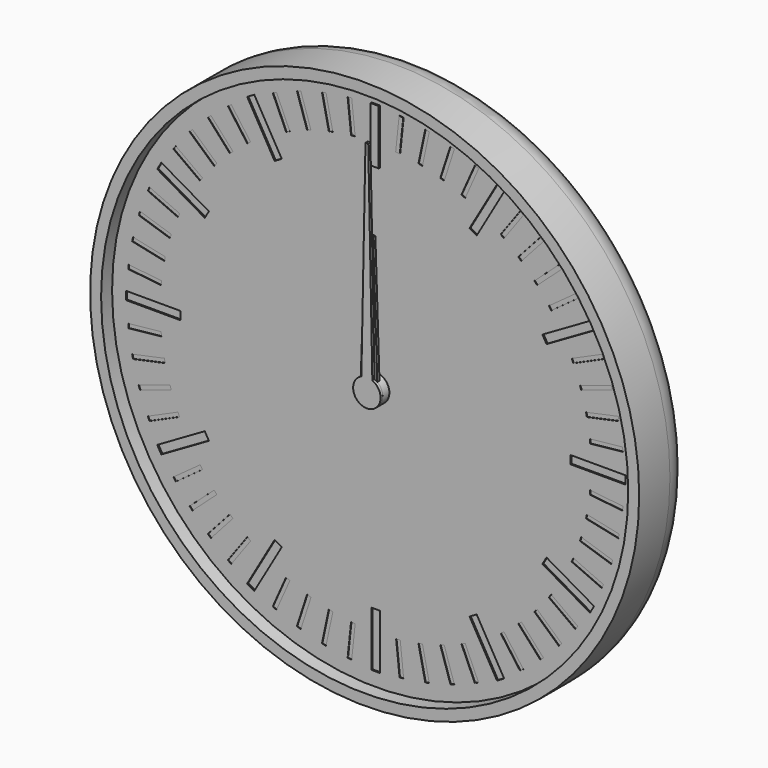
from build123d import *

# Parameters (mm, degrees)
F0_R      = 100
F1_DEPTH  = 24
F2_R      = 10
F3_T      = -4
F4_R      = 5
F4_R_2    = 3
F5_DEPTH  = 2
F6_DEPTH  = 19
F7_DEPTH  = 8
F9_DEPTH  = 4
F11_DEPTH = 4
F12_R     = 5
F12_R_2   = 3
F13_DEPTH = 2
F14_R     = 3
F15_DEPTH = 4
F17_DEPTH = 4
F18_R     = 3
F19_DEPTH = 2
F20_R     = 98
F20_R_2   = 5
F21_DEPTH = 1
F23_R     = 5
F23_R_2   = 3
F24_DEPTH = 2
F25_W     = 3
F25_H     = 20
F25_W_2   = 20
F25_H_2   = 3
F26_DEPTH = 0.5
F27_W     = 1.5
F27_H     = 12
F27_W_2   = 12
F27_H_2   = 1.5
F28_DEPTH = 0.2
F29_DEPTH = 1
F30_DEPTH = 0.4
F31_R     = 5
F31_R_2   = 3
F32_DEPTH = 5
F33_R     = 3
F34_DEPTH = 1
F36_DEPTH = 1


with BuildPart() as f1:
    # F0 (on Front) → F1 (new body)
    with BuildSketch(Plane.XZ):
        Circle(F0_R)
    extrude(amount=F1_DEPTH)

    # F2
    f2_edges = [f1.edges().sort_by_distance(p)[0] for p in [
        (-100, 0, 0),
    ]]
    fillet(f2_edges, radius=F2_R)

    # F3
    f3_openings = [f1.faces().sort_by_distance(p)[0] for p in [
        (0, -24, 0),
    ]]
    offset(amount=F3_T, openings=f3_openings)

    # F4 (on face) → F5 (join)
    with BuildSketch(Plane.XZ.offset(4)):
        Circle(F4_R)
        Circle(F4_R_2, mode=Mode.SUBTRACT)
        with Locations((40, 0)):
            Circle(F4_R)
        with Locations((40, 0)):
            Circle(F4_R_2, mode=Mode.SUBTRACT)
    extrude(amount=F5_DEPTH)


with BuildPart() as f6:
    # F6 (new): a face of the model
    f6_faces = [f1.part.faces().sort_by_distance(p)[0] for p in [
        (0, -4, 0),
    ]]
    extrude(f6_faces, amount=F6_DEPTH)

    # F8 (on face) → F9 (join)
    with BuildSketch(Plane.XZ.offset(6)):
        with BuildLine():
            ThreePointArc((9.2729637667, -1.3794085621), (9.3494561423, -0.6915886375), (9.375, 0))
            ThreePointArc((9.375, 0), (9.3494561423, 0.6915886375), (9.2729637667, 1.3794085621))
            ThreePointArc((9.2729637667, 1.3794085621), (8.9161548403, 2.8970343223), (8.3127812852, 4.3345463782))
            ThreePointArc((8.3127812852, 4.3345463782), (7.5845343223, 5.5104867402), (6.6911892658, 6.566476316))
            ThreePointArc((6.6911892658, 6.566476316), (5.5104867402, 7.5845343223), (4.1773988938, 8.3928519278))
            ThreePointArc((4.1773988938, 8.3928519278), (2.8970343223, 8.9161548403), (1.5536078905, 9.2453733036))
            ThreePointArc((1.5536078905, 9.2453733036), (0, 9.375), (-1.5536078905, 9.2453733036))
            ThreePointArc((-1.5536078905, 9.2453733036), (-2.8970343223, 8.9161548403), (-4.1773988938, 8.3928519278))
            ThreePointArc((-4.1773988938, 8.3928519278), (-5.5104867402, 7.5845343223), (-6.6911892658, 6.566476316))
            ThreePointArc((-6.6911892658, 6.566476316), (-7.5845343223, 5.5104867402), (-8.3127812852, 4.3345463782))
            ThreePointArc((-8.3127812852, 4.3345463782), (-8.9161548403, 2.8970343223), (-9.2729637667, 1.3794085621))
            ThreePointArc((-9.2729637667, 1.3794085621), (-9.375, 0), (-9.2729637667, -1.3794085621))
            ThreePointArc((-9.2729637667, -1.3794085621), (-8.9161548403, -2.8970343223), (-8.3127812852, -4.3345463782))
            ThreePointArc((-8.3127812852, -4.3345463782), (-7.5845343223, -5.5104867402), (-6.6911892658, -6.566476316))
            ThreePointArc((-6.6911892658, -6.566476316), (-5.5104867402, -7.5845343223), (-4.1773988938, -8.3928519278))
            ThreePointArc((-4.1773988938, -8.3928519278), (-2.8970343223, -8.9161548403), (-1.5536078905, -9.2453733036))
            ThreePointArc((-1.5536078905, -9.2453733036), (0, -9.375), (1.5536078905, -9.2453733036))
            ThreePointArc((1.5536078905, -9.2453733036), (2.8970343223, -8.9161548403), (4.1773988938, -8.3928519278))
            ThreePointArc((4.1773988938, -8.3928519278), (5.5104867402, -7.5845343223), (6.6911892658, -6.566476316))
            ThreePointArc((6.6911892658, -6.566476316), (7.5845343223, -5.5104867402), (8.3127812852, -4.3345463782))
            ThreePointArc((8.3127812852, -4.3345463782), (8.9161548403, -2.8970343223), (9.2729637667, -1.3794085621))
        make_face()
        with BuildLine():
            ThreePointArc((8.3127812852, 4.3345463782), (8.9161548403, 2.8970343223), (9.2729637667, 1.3794085621))
            Line((9.2729637667, 1.3794085621), (11.1823199426, 2.3946312492))
            Line((11.1823199426, 2.3946312492), (10.8182678729, 3.515068311))
            Line((10.8182678729, 3.515068311), (10.4542158031, 4.6355053728))
            Line((10.4542158031, 4.6355053728), (8.3127812852, 4.3345463782))
        make_face()
        with BuildLine():
            Line((11.1823199426, -2.3946312492), (9.2729637667, -1.3794085621))
            ThreePointArc((9.2729637667, -1.3794085621), (8.9161548403, -2.8970343223), (8.3127812852, -4.3345463782))
            Line((8.3127812852, -4.3345463782), (10.4542158031, -4.6355053728))
            Line((10.4542158031, -4.6355053728), (10.8182678729, -3.515068311))
            Line((10.8182678729, -3.515068311), (11.1823199426, -2.3946312492))
        make_face()
        with BuildLine():
            ThreePointArc((4.1773988938, 8.3928519278), (5.5104867402, 7.5845343223), (6.6911892658, 6.566476316))
            Line((6.6911892658, 6.566476316), (7.6391579371, 8.5101001246))
            Line((7.6391579371, 8.5101001246), (6.6860572448, 9.202568311))
            Line((6.6860572448, 9.202568311), (5.7329565525, 9.8950364974))
            Line((5.7329565525, 9.8950364974), (4.1773988938, 8.3928519278))
        make_face()
        with BuildLine():
            Line((7.6391579371, -8.5101001246), (6.6911892658, -6.566476316))
            ThreePointArc((6.6911892658, -6.566476316), (5.5104867402, -7.5845343223), (4.1773988938, -8.3928519278))
            Line((4.1773988938, -8.3928519278), (5.7329565525, -9.8950364974))
            Line((5.7329565525, -9.8950364974), (6.6860572448, -9.202568311))
            Line((6.6860572448, -9.202568311), (7.6391579371, -8.5101001246))
        make_face()
        with BuildLine():
            ThreePointArc((-1.5536078905, 9.2453733036), (0, 9.375), (1.5536078905, 9.2453733036))
            Line((1.5536078905, 9.2453733036), (1.1780972451, 11.375))
            Line((1.1780972451, 11.375), (0, 11.375))
            Line((0, 11.375), (-1.1780972451, 11.375))
            Line((-1.1780972451, 11.375), (-1.5536078905, 9.2453733036))
        make_face()
        with BuildLine():
            Line((1.1780972451, -11.375), (1.5536078905, -9.2453733036))
            ThreePointArc((1.5536078905, -9.2453733036), (0, -9.375), (-1.5536078905, -9.2453733036))
            Line((-1.5536078905, -9.2453733036), (-1.1780972451, -11.375))
            Line((-1.1780972451, -11.375), (0, -11.375))
            Line((0, -11.375), (1.1780972451, -11.375))
        make_face()
        with BuildLine():
            ThreePointArc((-6.6911892658, 6.566476316), (-5.5104867402, 7.5845343223), (-4.1773988938, 8.3928519278))
            Line((-4.1773988938, 8.3928519278), (-5.7329565525, 9.8950364974))
            Line((-5.7329565525, 9.8950364974), (-6.6860572448, 9.202568311))
            Line((-6.6860572448, 9.202568311), (-7.6391579371, 8.5101001246))
            Line((-7.6391579371, 8.5101001246), (-6.6911892658, 6.566476316))
        make_face()
        with BuildLine():
            Line((-5.7329565525, -9.8950364974), (-4.1773988938, -8.3928519278))
            ThreePointArc((-4.1773988938, -8.3928519278), (-5.5104867402, -7.5845343223), (-6.6911892658, -6.566476316))
            Line((-6.6911892658, -6.566476316), (-7.6391579371, -8.5101001246))
            Line((-7.6391579371, -8.5101001246), (-6.6860572448, -9.202568311))
            Line((-6.6860572448, -9.202568311), (-5.7329565525, -9.8950364974))
        make_face()
        with BuildLine():
            ThreePointArc((-9.2729637667, 1.3794085621), (-8.9161548403, 2.8970343223), (-8.3127812852, 4.3345463782))
            Line((-8.3127812852, 4.3345463782), (-10.4542158031, 4.6355053728))
            Line((-10.4542158031, 4.6355053728), (-10.8182678729, 3.515068311))
            Line((-10.8182678729, 3.515068311), (-11.1823199426, 2.3946312492))
            Line((-11.1823199426, 2.3946312492), (-9.2729637667, 1.3794085621))
        make_face()
        with BuildLine():
            Line((-10.4542158031, -4.6355053728), (-8.3127812852, -4.3345463782))
            ThreePointArc((-8.3127812852, -4.3345463782), (-8.9161548403, -2.8970343223), (-9.2729637667, -1.3794085621))
            Line((-9.2729637667, -1.3794085621), (-11.1823199426, -2.3946312492))
            Line((-11.1823199426, -2.3946312492), (-10.8182678729, -3.515068311))
            Line((-10.8182678729, -3.515068311), (-10.4542158031, -4.6355053728))
        make_face()
    extrude(amount=F9_DEPTH)

    # F35 (on face) → F36 (join)
    with BuildSketch(Plane.XZ.offset(23)):
        with BuildLine():
            ThreePointArc((-2, 4.582575695), (-2.7386127875, -4.1833001327), (5, 0))
            ThreePointArc((5, 0), (4.1833001327, 2.7386127875), (2, 4.582575695))
            ThreePointArc((2, 4.582575695), (0, 5), (-2, 4.582575695))
        make_face()
        with BuildLine():
            ThreePointArc((-2, 4.582575695), (0, 5), (2, 4.582575695))
            Line((2, 4.582575695), (0.5, 80))
            Line((0.5, 80), (0, 80))
            Line((0, 80), (-0.5, 80))
            Line((-0.5, 80), (-2, 4.582575695))
        make_face()
    extrude(amount=-F36_DEPTH)


with BuildPart() as f7:
    # F7 (new): a face of the model
    f7_faces = [f1.part.faces().sort_by_distance(p)[0] for p in [
        (40, -4, 0),
    ]]
    extrude(f7_faces, amount=F7_DEPTH)

    # F10 (on face) → F11 (join)
    with BuildSketch(Plane.XZ.offset(6)):
        with BuildLine():
            ThreePointArc((68.0829066802, -1.5381733945), (68.1144747006, -0.7693746225), (68.125, 0))
            ThreePointArc((68.125, 0), (68.1144747006, 0.7693746225), (68.0829066802, 1.5381733945))
            ThreePointArc((68.0829066802, 1.5381733945), (67.9709283072, 2.9398630294), (67.7890320221, 4.3342039956))
            ThreePointArc((67.7890320221, 4.3342039956), (67.5104012706, 5.8475163042), (67.1494235596, 7.3433252263))
            ThreePointArc((67.1494235596, 7.3433252263), (66.7484645208, 8.6911029668), (66.280643318, 10.0171558733))
            ThreePointArc((66.280643318, 10.0171558733), (65.6934659962, 11.4394680865), (65.0293803521, 12.8275385085))
            ThreePointArc((65.0293803521, 12.8275385085), (64.3569644814, 14.0625), (63.6236643925, 15.2623099717))
            ThreePointArc((63.6236643925, 15.2623099717), (62.7536029668, 16.5314602207), (61.815433119, 17.7511268046))
            ThreePointArc((61.815433119, 17.7511268046), (60.9009482166, 18.8192983038), (59.934217974, 19.8404278876))
            ThreePointArc((59.934217974, 19.8404278876), (58.8192983038, 20.9009482166), (57.6480467764, 21.8989056799))
            ThreePointArc((57.6480467764, 21.8989056799), (56.5314602207, 22.7536029668), (55.3735505752, 23.5514238999))
            ThreePointArc((55.3735505752, 23.5514238999), (54.0625, 24.3569644814), (52.709356105, 25.0895972944))
            ThreePointArc((52.709356105, 25.0895972944), (51.4394680865, 25.6934659962), (50.1409852457, 26.2331096755))
            ThreePointArc((50.1409852457, 26.2331096755), (48.6911029668, 26.7484645208), (47.2152055856, 27.1837531139))
            ThreePointArc((47.2152055856, 27.1837531139), (45.8475163042, 27.5104012706), (44.4652101991, 27.7682826779))
            ThreePointArc((44.4652101991, 27.7682826779), (42.9398630294, 27.9709283072), (41.4057159597, 28.0898484802))
            ThreePointArc((41.4057159597, 28.0898484802), (40, 28.125), (38.5942840403, 28.0898484802))
            ThreePointArc((38.5942840403, 28.0898484802), (37.0601369706, 27.9709283072), (35.5347898009, 27.7682826779))
            ThreePointArc((35.5347898009, 27.7682826779), (34.1524836958, 27.5104012706), (32.7847944144, 27.1837531139))
            ThreePointArc((32.7847944144, 27.1837531139), (31.3088970332, 26.7484645208), (29.8590147543, 26.2331096755))
            ThreePointArc((29.8590147543, 26.2331096755), (28.5605319135, 25.6934659962), (27.290643895, 25.0895972944))
            ThreePointArc((27.290643895, 25.0895972944), (25.9375, 24.3569644814), (24.6264494248, 23.5514238999))
            ThreePointArc((24.6264494248, 23.5514238999), (23.4685397793, 22.7536029668), (22.3519532236, 21.8989056799))
            ThreePointArc((22.3519532236, 21.8989056799), (21.1807016962, 20.9009482166), (20.065782026, 19.8404278876))
            ThreePointArc((20.065782026, 19.8404278876), (19.0990517834, 18.8192983038), (18.184566881, 17.7511268046))
            ThreePointArc((18.184566881, 17.7511268046), (17.2463970332, 16.5314602207), (16.3763356075, 15.2623099717))
            ThreePointArc((16.3763356075, 15.2623099717), (15.6430355186, 14.0625), (14.9706196479, 12.8275385085))
            ThreePointArc((14.9706196479, 12.8275385085), (14.3065340038, 11.4394680865), (13.719356682, 10.0171558733))
            ThreePointArc((13.719356682, 10.0171558733), (13.2515354792, 8.6911029668), (12.8505764404, 7.3433252263))
            ThreePointArc((12.8505764404, 7.3433252263), (12.4895987294, 5.8475163042), (12.2109679779, 4.3342039956))
            ThreePointArc((12.2109679779, 4.3342039956), (12.0290716928, 2.9398630294), (11.9170933198, 1.5381733945))
            ThreePointArc((11.9170933198, 1.5381733945), (11.875, 0), (11.9170933198, -1.5381733945))
            ThreePointArc((11.9170933198, -1.5381733945), (12.0290716928, -2.9398630294), (12.2109679779, -4.3342039956))
            ThreePointArc((12.2109679779, -4.3342039956), (12.4895987294, -5.8475163042), (12.8505764404, -7.3433252263))
            ThreePointArc((12.8505764404, -7.3433252263), (13.2515354792, -8.6911029668), (13.719356682, -10.0171558733))
            ThreePointArc((13.719356682, -10.0171558733), (14.3065340038, -11.4394680865), (14.9706196479, -12.8275385085))
            ThreePointArc((14.9706196479, -12.8275385085), (15.6430355186, -14.0625), (16.3763356075, -15.2623099717))
            ThreePointArc((16.3763356075, -15.2623099717), (17.2463970332, -16.5314602207), (18.184566881, -17.7511268046))
            ThreePointArc((18.184566881, -17.7511268046), (19.0990517834, -18.8192983038), (20.065782026, -19.8404278876))
            ThreePointArc((20.065782026, -19.8404278876), (21.1807016962, -20.9009482166), (22.3519532236, -21.8989056799))
            ThreePointArc((22.3519532236, -21.8989056799), (23.4685397793, -22.7536029668), (24.6264494248, -23.5514238999))
            ThreePointArc((24.6264494248, -23.5514238999), (25.9375, -24.3569644814), (27.290643895, -25.0895972944))
            ThreePointArc((27.290643895, -25.0895972944), (28.5605319135, -25.6934659962), (29.8590147543, -26.2331096755))
            ThreePointArc((29.8590147543, -26.2331096755), (31.3088970332, -26.7484645208), (32.7847944144, -27.1837531139))
            ThreePointArc((32.7847944144, -27.1837531139), (34.1524836958, -27.5104012706), (35.5347898009, -27.7682826779))
            ThreePointArc((35.5347898009, -27.7682826779), (37.0601369706, -27.9709283072), (38.5942840403, -28.0898484802))
            ThreePointArc((38.5942840403, -28.0898484802), (40, -28.125), (41.4057159597, -28.0898484802))
            ThreePointArc((41.4057159597, -28.0898484802), (42.9398630294, -27.9709283072), (44.4652101991, -27.7682826779))
            ThreePointArc((44.4652101991, -27.7682826779), (45.8475163042, -27.5104012706), (47.2152055856, -27.1837531139))
            ThreePointArc((47.2152055856, -27.1837531139), (48.6911029668, -26.7484645208), (50.1409852457, -26.2331096755))
            ThreePointArc((50.1409852457, -26.2331096755), (51.4394680865, -25.6934659962), (52.709356105, -25.0895972944))
            ThreePointArc((52.709356105, -25.0895972944), (54.0625, -24.3569644814), (55.3735505752, -23.5514238999))
            ThreePointArc((55.3735505752, -23.5514238999), (56.5314602207, -22.7536029668), (57.6480467764, -21.8989056799))
            ThreePointArc((57.6480467764, -21.8989056799), (58.8192983038, -20.9009482166), (59.934217974, -19.8404278876))
            ThreePointArc((59.934217974, -19.8404278876), (60.9009482166, -18.8192983038), (61.815433119, -17.7511268046))
            ThreePointArc((61.815433119, -17.7511268046), (62.7536029668, -16.5314602207), (63.6236643925, -15.2623099717))
            ThreePointArc((63.6236643925, -15.2623099717), (64.3569644814, -14.0625), (65.0293803521, -12.8275385085))
            ThreePointArc((65.0293803521, -12.8275385085), (65.6934659962, -11.4394680865), (66.280643318, -10.0171558733))
            ThreePointArc((66.280643318, -10.0171558733), (66.7484645208, -8.6911029668), (67.1494235596, -7.3433252263))
            ThreePointArc((67.1494235596, -7.3433252263), (67.5104012706, -5.8475163042), (67.7890320221, -4.3342039956))
            ThreePointArc((67.7890320221, -4.3342039956), (67.9709283072, -2.9398630294), (68.0829066802, -1.5381733945))
        make_face()
        with BuildLine():
            ThreePointArc((68.0829066802, 1.5381733945), (68.1144747006, 0.7693746225), (68.125, 0))
            ThreePointArc((68.125, 0), (68.1144747006, -0.7693746225), (68.0829066802, -1.5381733945))
            Line((68.0829066802, -1.5381733945), (70.125, -1.1780972451))
            Line((70.125, -1.1780972451), (70.125, 0))
            Line((70.125, 0), (70.125, 1.1780972451))
            Line((70.125, 1.1780972451), (68.0829066802, 1.5381733945))
        make_face()
        with BuildLine():
            ThreePointArc((67.1494235596, 7.3433252263), (67.5104012706, 5.8475163042), (67.7890320221, 4.3342039956))
            Line((67.7890320221, 4.3342039956), (69.7116366623, 5.1109866922))
            Line((69.7116366623, 5.1109866922), (69.4666964721, 6.2633396859))
            Line((69.4666964721, 6.2633396859), (69.2217562819, 7.4156926796))
            Line((69.2217562819, 7.4156926796), (67.1494235596, 7.3433252263))
        make_face()
        with BuildLine():
            Line((69.7116366623, -5.1109866922), (67.7890320221, -4.3342039956))
            ThreePointArc((67.7890320221, -4.3342039956), (67.5104012706, -5.8475163042), (67.1494235596, -7.3433252263))
            Line((67.1494235596, -7.3433252263), (69.2217562819, -7.4156926796))
            Line((69.2217562819, -7.4156926796), (69.4666964721, -6.2633396859))
            Line((69.4666964721, -6.2633396859), (69.7116366623, -5.1109866922))
        make_face()
        with BuildLine():
            ThreePointArc((65.0293803521, 12.8275385085), (65.6934659962, 11.4394680865), (66.280643318, 10.0171558733))
            Line((66.280643318, 10.0171558733), (67.9997322302, 11.1766959857))
            Line((67.9997322302, 11.1766959857), (67.5205569115, 12.2529413727))
            Line((67.5205569115, 12.2529413727), (67.0413815928, 13.3291867596))
            Line((67.0413815928, 13.3291867596), (65.0293803521, 12.8275385085))
        make_face()
        with BuildLine():
            Line((67.9997322302, -11.1766959857), (66.280643318, -10.0171558733))
            ThreePointArc((66.280643318, -10.0171558733), (65.6934659962, -11.4394680865), (65.0293803521, -12.8275385085))
            Line((65.0293803521, -12.8275385085), (67.0413815928, -13.3291867596))
            Line((67.0413815928, -13.3291867596), (67.5205569115, -12.2529413727))
            Line((67.5205569115, -12.2529413727), (67.9997322302, -11.1766959857))
        make_face()
        with BuildLine():
            ThreePointArc((61.815433119, 17.7511268046), (62.7536029668, 16.5314602207), (63.6236643925, 15.2623099717))
            Line((63.6236643925, 15.2623099717), (65.064105142, 16.753930033))
            Line((65.064105142, 16.753930033), (64.3716369555, 17.7070307253))
            Line((64.3716369555, 17.7070307253), (63.6791687691, 18.6601314176))
            Line((63.6791687691, 18.6601314176), (61.815433119, 17.7511268046))
        make_face()
        with BuildLine():
            Line((65.064105142, -16.753930033), (63.6236643925, -15.2623099717))
            ThreePointArc((63.6236643925, -15.2623099717), (62.7536029668, -16.5314602207), (61.815433119, -17.7511268046))
            Line((61.815433119, -17.7511268046), (63.6791687691, -18.6601314176))
            Line((63.6791687691, -18.6601314176), (64.3716369555, -17.7070307253))
            Line((64.3716369555, -17.7070307253), (65.064105142, -16.753930033))
        make_face()
        with BuildLine():
            ThreePointArc((57.6480467764, 21.8989056799), (58.8192983038, 20.9009482166), (59.934217974, 19.8404278876))
            Line((59.934217974, 19.8404278876), (61.0330563882, 21.5989369435))
            Line((61.0330563882, 21.5989369435), (60.1575595166, 22.3872378675))
            Line((60.1575595166, 22.3872378675), (59.282062645, 23.1755387915))
            Line((59.282062645, 23.1755387915), (57.6480467764, 21.8989056799))
        make_face()
        with BuildLine():
            Line((61.0330563882, -21.5989369435), (59.934217974, -19.8404278876))
            ThreePointArc((59.934217974, -19.8404278876), (58.8192983038, -20.9009482166), (57.6480467764, -21.8989056799))
            Line((57.6480467764, -21.8989056799), (59.282062645, -23.1755387915))
            Line((59.282062645, -23.1755387915), (60.1575595166, -22.3872378675))
            Line((60.1575595166, -22.3872378675), (61.0330563882, -21.5989369435))
        make_face()
        with BuildLine():
            ThreePointArc((52.709356105, 25.0895972944), (54.0625, 24.3569644814), (55.3735505752, 23.5514238999))
            Line((55.3735505752, 23.5514238999), (56.0827621424, 25.4999666665))
            Line((56.0827621424, 25.4999666665), (55.0625, 26.089015289))
            Line((55.0625, 26.089015289), (54.0422378576, 26.6780639116))
            Line((54.0422378576, 26.6780639116), (52.709356105, 25.0895972944))
        make_face()
        with BuildLine():
            Line((56.0827621424, -25.4999666665), (55.3735505752, -23.5514238999))
            ThreePointArc((55.3735505752, -23.5514238999), (54.0625, -24.3569644814), (52.709356105, -25.0895972944))
            Line((52.709356105, -25.0895972944), (54.0422378576, -26.6780639116))
            Line((54.0422378576, -26.6780639116), (55.0625, -26.089015289))
            Line((55.0625, -26.089015289), (56.0827621424, -25.4999666665))
        make_face()
        with BuildLine():
            ThreePointArc((47.2152055856, 27.1837531139), (48.6911029668, 26.7484645208), (50.1409852457, 26.2331096755))
            Line((50.1409852457, 26.2331096755), (50.4295740173, 28.2865254836))
            Line((50.4295740173, 28.2865254836), (49.3091369555, 28.6505775534))
            Line((49.3091369555, 28.6505775534), (48.1886998938, 29.0146296232))
            Line((48.1886998938, 29.0146296232), (47.2152055856, 27.1837531139))
        make_face()
        with BuildLine():
            Line((50.4295740173, -28.2865254836), (50.1409852457, -26.2331096755))
            ThreePointArc((50.1409852457, -26.2331096755), (48.6911029668, -26.7484645208), (47.2152055856, -27.1837531139))
            Line((47.2152055856, -27.1837531139), (48.1886998938, -29.0146296232))
            Line((48.1886998938, -29.0146296232), (49.3091369555, -28.6505775534))
            Line((49.3091369555, -28.6505775534), (50.4295740173, -28.2865254836))
        make_face()
        with BuildLine():
            ThreePointArc((41.4057159597, 28.0898484802), (42.9398630294, 27.9709283072), (44.4652101991, 27.7682826779))
            Line((44.4652101991, 27.7682826779), (44.3205634611, 29.8368274034))
            Line((44.3205634611, 29.8368274034), (43.1489199559, 29.959972098))
            Line((43.1489199559, 29.959972098), (41.9772764508, 30.0831167926))
            Line((41.9772764508, 30.0831167926), (41.4057159597, 28.0898484802))
        make_face()
        with BuildLine():
            Line((44.3205634611, -29.8368274034), (44.4652101991, -27.7682826779))
            ThreePointArc((44.4652101991, -27.7682826779), (42.9398630294, -27.9709283072), (41.4057159597, -28.0898484802))
            Line((41.4057159597, -28.0898484802), (41.9772764508, -30.0831167926))
            Line((41.9772764508, -30.0831167926), (43.1489199559, -29.959972098))
            Line((43.1489199559, -29.959972098), (44.3205634611, -29.8368274034))
        make_face()
        with BuildLine():
            ThreePointArc((35.5347898009, 27.7682826779), (37.0601369706, 27.9709283072), (38.5942840403, 28.0898484802))
            Line((38.5942840403, 28.0898484802), (38.0227235492, 30.0831167926))
            Line((38.0227235492, 30.0831167926), (36.8510800441, 29.959972098))
            Line((36.8510800441, 29.959972098), (35.6794365389, 29.8368274034))
            Line((35.6794365389, 29.8368274034), (35.5347898009, 27.7682826779))
        make_face()
        with BuildLine():
            Line((38.0227235492, -30.0831167926), (38.5942840403, -28.0898484802))
            ThreePointArc((38.5942840403, -28.0898484802), (37.0601369706, -27.9709283072), (35.5347898009, -27.7682826779))
            Line((35.5347898009, -27.7682826779), (35.6794365389, -29.8368274034))
            Line((35.6794365389, -29.8368274034), (36.8510800441, -29.959972098))
            Line((36.8510800441, -29.959972098), (38.0227235492, -30.0831167926))
        make_face()
        with BuildLine():
            ThreePointArc((29.8590147543, 26.2331096755), (31.3088970332, 26.7484645208), (32.7847944144, 27.1837531139))
            Line((32.7847944144, 27.1837531139), (31.8113001062, 29.0146296232))
            Line((31.8113001062, 29.0146296232), (30.6908630445, 28.6505775534))
            Line((30.6908630445, 28.6505775534), (29.5704259827, 28.2865254836))
            Line((29.5704259827, 28.2865254836), (29.8590147543, 26.2331096755))
        make_face()
        with BuildLine():
            Line((31.8113001062, -29.0146296232), (32.7847944144, -27.1837531139))
            ThreePointArc((32.7847944144, -27.1837531139), (31.3088970332, -26.7484645208), (29.8590147543, -26.2331096755))
            Line((29.8590147543, -26.2331096755), (29.5704259827, -28.2865254836))
            Line((29.5704259827, -28.2865254836), (30.6908630445, -28.6505775534))
            Line((30.6908630445, -28.6505775534), (31.8113001062, -29.0146296232))
        make_face()
        with BuildLine():
            ThreePointArc((24.6264494248, 23.5514238999), (25.9375, 24.3569644814), (27.290643895, 25.0895972944))
            Line((27.290643895, 25.0895972944), (25.9577621424, 26.6780639116))
            Line((25.9577621424, 26.6780639116), (24.9375, 26.089015289))
            Line((24.9375, 26.089015289), (23.9172378576, 25.4999666665))
            Line((23.9172378576, 25.4999666665), (24.6264494248, 23.5514238999))
        make_face()
        with BuildLine():
            Line((25.9577621424, -26.6780639116), (27.290643895, -25.0895972944))
            ThreePointArc((27.290643895, -25.0895972944), (25.9375, -24.3569644814), (24.6264494248, -23.5514238999))
            Line((24.6264494248, -23.5514238999), (23.9172378576, -25.4999666665))
            Line((23.9172378576, -25.4999666665), (24.9375, -26.089015289))
            Line((24.9375, -26.089015289), (25.9577621424, -26.6780639116))
        make_face()
        with BuildLine():
            ThreePointArc((20.065782026, 19.8404278876), (21.1807016962, 20.9009482166), (22.3519532236, 21.8989056799))
            Line((22.3519532236, 21.8989056799), (20.717937355, 23.1755387915))
            Line((20.717937355, 23.1755387915), (19.8424404834, 22.3872378675))
            Line((19.8424404834, 22.3872378675), (18.9669436118, 21.5989369435))
            Line((18.9669436118, 21.5989369435), (20.065782026, 19.8404278876))
        make_face()
        with BuildLine():
            Line((20.717937355, -23.1755387915), (22.3519532236, -21.8989056799))
            ThreePointArc((22.3519532236, -21.8989056799), (21.1807016962, -20.9009482166), (20.065782026, -19.8404278876))
            Line((20.065782026, -19.8404278876), (18.9669436118, -21.5989369435))
            Line((18.9669436118, -21.5989369435), (19.8424404834, -22.3872378675))
            Line((19.8424404834, -22.3872378675), (20.717937355, -23.1755387915))
        make_face()
        with BuildLine():
            ThreePointArc((16.3763356075, 15.2623099717), (17.2463970332, 16.5314602207), (18.184566881, 17.7511268046))
            Line((18.184566881, 17.7511268046), (16.3208312309, 18.6601314176))
            Line((16.3208312309, 18.6601314176), (15.6283630445, 17.7070307253))
            Line((15.6283630445, 17.7070307253), (14.935894858, 16.753930033))
            Line((14.935894858, 16.753930033), (16.3763356075, 15.2623099717))
        make_face()
        with BuildLine():
            Line((16.3208312309, -18.6601314176), (18.184566881, -17.7511268046))
            ThreePointArc((18.184566881, -17.7511268046), (17.2463970332, -16.5314602207), (16.3763356075, -15.2623099717))
            Line((16.3763356075, -15.2623099717), (14.935894858, -16.753930033))
            Line((14.935894858, -16.753930033), (15.6283630445, -17.7070307253))
            Line((15.6283630445, -17.7070307253), (16.3208312309, -18.6601314176))
        make_face()
        with BuildLine():
            ThreePointArc((13.719356682, 10.0171558733), (14.3065340038, 11.4394680865), (14.9706196479, 12.8275385085))
            Line((14.9706196479, 12.8275385085), (12.9586184072, 13.3291867596))
            Line((12.9586184072, 13.3291867596), (12.4794430885, 12.2529413727))
            Line((12.4794430885, 12.2529413727), (12.0002677698, 11.1766959857))
            Line((12.0002677698, 11.1766959857), (13.719356682, 10.0171558733))
        make_face()
        with BuildLine():
            Line((12.9586184072, -13.3291867596), (14.9706196479, -12.8275385085))
            ThreePointArc((14.9706196479, -12.8275385085), (14.3065340038, -11.4394680865), (13.719356682, -10.0171558733))
            Line((13.719356682, -10.0171558733), (12.0002677698, -11.1766959857))
            Line((12.0002677698, -11.1766959857), (12.4794430885, -12.2529413727))
            Line((12.4794430885, -12.2529413727), (12.9586184072, -13.3291867596))
        make_face()
        with BuildLine():
            ThreePointArc((12.2109679779, 4.3342039956), (12.4895987294, 5.8475163042), (12.8505764404, 7.3433252263))
            Line((12.8505764404, 7.3433252263), (10.7782437181, 7.4156926796))
            Line((10.7782437181, 7.4156926796), (10.5333035279, 6.2633396859))
            Line((10.5333035279, 6.2633396859), (10.2883633377, 5.1109866922))
            Line((10.2883633377, 5.1109866922), (12.2109679779, 4.3342039956))
        make_face()
        with BuildLine():
            Line((10.7782437181, -7.4156926796), (12.8505764404, -7.3433252263))
            ThreePointArc((12.8505764404, -7.3433252263), (12.4895987294, -5.8475163042), (12.2109679779, -4.3342039956))
            Line((12.2109679779, -4.3342039956), (10.2883633377, -5.1109866922))
            Line((10.2883633377, -5.1109866922), (10.5333035279, -6.2633396859))
            Line((10.5333035279, -6.2633396859), (10.7782437181, -7.4156926796))
        make_face()
        with BuildLine():
            ThreePointArc((11.9170933198, -1.5381733945), (11.875, 0), (11.9170933198, 1.5381733945))
            Line((11.9170933198, 1.5381733945), (9.875, 1.1780972451))
            Line((9.875, 1.1780972451), (9.875, 0))
            Line((9.875, 0), (9.875, -1.1780972451))
            Line((9.875, -1.1780972451), (11.9170933198, -1.5381733945))
        make_face()
    extrude(amount=F11_DEPTH)

    # F16 (on face) → F17 (join)
    with BuildSketch(Plane.XZ.offset(12)):
        with BuildLine():
            ThreePointArc((47.4288750323, -1.0304444454), (47.4821976298, -0.5164480894), (47.5, 0))
            ThreePointArc((47.5, 0), (47.4821976298, 0.5164480894), (47.4288750323, 1.0304444454))
            ThreePointArc((47.4288750323, 1.0304444454), (47.1329238722, 2.3176274578), (46.6157661985, 3.532936117))
            ThreePointArc((46.6157661985, 3.532936117), (46.0676274578, 4.4083893922), (45.4044061018, 5.2002302532))
            ThreePointArc((45.4044061018, 5.2002302532), (44.4083893922, 6.0676274578), (43.2756595386, 6.7468551628))
            ThreePointArc((43.2756595386, 6.7468551628), (42.3176274578, 7.1329238722), (41.3156377295, 7.3837048536))
            ThreePointArc((41.3156377295, 7.3837048536), (40, 7.5), (38.6843622705, 7.3837048536))
            ThreePointArc((38.6843622705, 7.3837048536), (37.6823725422, 7.1329238722), (36.7243404614, 6.7468551628))
            ThreePointArc((36.7243404614, 6.7468551628), (35.5916106078, 6.0676274578), (34.5955938982, 5.2002302532))
            ThreePointArc((34.5955938982, 5.2002302532), (33.9323725422, 4.4083893922), (33.3842338015, 3.532936117))
            ThreePointArc((33.3842338015, 3.532936117), (32.8670761278, 2.3176274578), (32.5711249677, 1.0304444454))
            ThreePointArc((32.5711249677, 1.0304444454), (32.5, 0), (32.5711249677, -1.0304444454))
            ThreePointArc((32.5711249677, -1.0304444454), (32.8670761278, -2.3176274578), (33.3842338015, -3.532936117))
            ThreePointArc((33.3842338015, -3.532936117), (33.9323725422, -4.4083893922), (34.5955938982, -5.2002302532))
            ThreePointArc((34.5955938982, -5.2002302532), (35.5916106078, -6.0676274578), (36.7243404614, -6.7468551628))
            ThreePointArc((36.7243404614, -6.7468551628), (37.6823725422, -7.1329238722), (38.6843622705, -7.3837048536))
            ThreePointArc((38.6843622705, -7.3837048536), (40, -7.5), (41.3156377295, -7.3837048536))
            ThreePointArc((41.3156377295, -7.3837048536), (42.3176274578, -7.1329238722), (43.2756595386, -6.7468551628))
            ThreePointArc((43.2756595386, -6.7468551628), (44.4083893922, -6.0676274578), (45.4044061018, -5.2002302532))
            ThreePointArc((45.4044061018, -5.2002302532), (46.0676274578, -4.4083893922), (46.6157661985, -3.532936117))
            ThreePointArc((46.6157661985, -3.532936117), (47.1329238722, -2.3176274578), (47.4288750323, -1.0304444454))
        make_face()
        with BuildLine():
            ThreePointArc((46.6157661985, 3.532936117), (47.1329238722, 2.3176274578), (47.4288750323, 1.0304444454))
            Line((47.4288750323, 1.0304444454), (49.3262785606, 2.0393117971))
            Line((49.3262785606, 2.0393117971), (48.743795249, 3.832011096))
            Line((48.743795249, 3.832011096), (46.6157661985, 3.532936117))
        make_face()
        with BuildLine():
            Line((49.3262785606, -2.0393117971), (47.4288750323, -1.0304444454))
            ThreePointArc((47.4288750323, -1.0304444454), (47.1329238722, -2.3176274578), (46.6157661985, -3.532936117))
            Line((46.6157661985, -3.532936117), (48.743795249, -3.832011096))
            Line((48.743795249, -3.832011096), (49.3262785606, -2.0393117971))
        make_face()
        with BuildLine():
            ThreePointArc((43.2756595386, 6.7468551628), (44.4083893922, 6.0676274578), (45.4044061018, 5.2002302532))
            Line((45.4044061018, 5.2002302532), (46.3464404506, 7.1316868974))
            Line((46.3464404506, 7.1316868974), (44.8214793429, 8.2396359957))
            Line((44.8214793429, 8.2396359957), (43.2756595386, 6.7468551628))
        make_face()
        with BuildLine():
            Line((46.3464404506, -7.1316868974), (45.4044061018, -5.2002302532))
            ThreePointArc((45.4044061018, -5.2002302532), (44.4083893922, -6.0676274578), (43.2756595386, -6.7468551628))
            Line((43.2756595386, -6.7468551628), (44.8214793429, -8.2396359957))
            Line((44.8214793429, -8.2396359957), (46.3464404506, -7.1316868974))
        make_face()
        with BuildLine():
            ThreePointArc((38.6843622705, 7.3837048536), (40, 7.5), (41.3156377295, 7.3837048536))
            Line((41.3156377295, 7.3837048536), (40.9424777961, 9.5))
            Line((40.9424777961, 9.5), (39.0575222039, 9.5))
            Line((39.0575222039, 9.5), (38.6843622705, 7.3837048536))
        make_face()
        with BuildLine():
            Line((40.9424777961, -9.5), (41.3156377295, -7.3837048536))
            ThreePointArc((41.3156377295, -7.3837048536), (40, -7.5), (38.6843622705, -7.3837048536))
            Line((38.6843622705, -7.3837048536), (39.0575222039, -9.5))
            Line((39.0575222039, -9.5), (40.9424777961, -9.5))
        make_face()
        with BuildLine():
            ThreePointArc((34.5955938982, 5.2002302532), (35.5916106078, 6.0676274578), (36.7243404614, 6.7468551628))
            Line((36.7243404614, 6.7468551628), (35.1785206571, 8.2396359957))
            Line((35.1785206571, 8.2396359957), (33.6535595494, 7.1316868974))
            Line((33.6535595494, 7.1316868974), (34.5955938982, 5.2002302532))
        make_face()
        with BuildLine():
            Line((35.1785206571, -8.2396359957), (36.7243404614, -6.7468551628))
            ThreePointArc((36.7243404614, -6.7468551628), (35.5916106078, -6.0676274578), (34.5955938982, -5.2002302532))
            Line((34.5955938982, -5.2002302532), (33.6535595494, -7.1316868974))
            Line((33.6535595494, -7.1316868974), (35.1785206571, -8.2396359957))
        make_face()
        with BuildLine():
            ThreePointArc((32.5711249677, 1.0304444454), (32.8670761278, 2.3176274578), (33.3842338015, 3.532936117))
            Line((33.3842338015, 3.532936117), (31.256204751, 3.832011096))
            Line((31.256204751, 3.832011096), (30.6737214394, 2.0393117971))
            Line((30.6737214394, 2.0393117971), (32.5711249677, 1.0304444454))
        make_face()
        with BuildLine():
            Line((31.256204751, -3.832011096), (33.3842338015, -3.532936117))
            ThreePointArc((33.3842338015, -3.532936117), (32.8670761278, -2.3176274578), (32.5711249677, -1.0304444454))
            Line((32.5711249677, -1.0304444454), (30.6737214394, -2.0393117971))
            Line((30.6737214394, -2.0393117971), (31.256204751, -3.832011096))
        make_face()
    extrude(amount=F17_DEPTH)

    # F18 (on face) → F19 (join)
    with BuildSketch(Plane.XZ.offset(16)):
        with Locations((40, 0)):
            Circle(F18_R)
    extrude(amount=F19_DEPTH)


with BuildPart() as f13:
    # F12 (on face) → F13 (new body)
    with BuildSketch(Plane.XZ.offset(10)):
        Circle(F12_R)
        Circle(F12_R_2, mode=Mode.SUBTRACT)
    extrude(amount=F13_DEPTH)

    # F14 (on face) → F15 (join)
    with BuildSketch(Plane.XZ.offset(12)):
        with BuildLine():
            ThreePointArc((29.9718156995, -1.3001014101), (29.9929530972, -0.6502034357), (30, 0))
            ThreePointArc((30, 0), (29.9929530972, 0.6502034357), (29.9718156995, 1.3001014101))
            ThreePointArc((29.9718156995, 1.3001014101), (29.907520012, 2.3537728718), (29.8061935814, 3.4045299509))
            ThreePointArc((29.8061935814, 3.4045299509), (29.6306502179, 4.6930339512), (29.3994322443, 5.9727199596))
            ThreePointArc((29.3994322443, 5.9727199596), (29.1710976119, 7.0033609157), (28.9066440563, 8.0253304855))
            ThreePointArc((28.9066440563, 8.0253304855), (28.5316954889, 9.2705098312), (28.1031371961, 10.4982703213))
            ThreePointArc((28.1031371961, 10.4982703213), (27.7163859753, 11.480502971), (27.2953170189, 12.448520749))
            ThreePointArc((27.2953170189, 12.448520749), (26.7301957257, 13.6197149922), (26.1148496411, 14.765318426))
            ThreePointArc((26.1148496411, 14.765318426), (25.5792049306, 15.6749569415), (25.0118886885, 16.5651871174))
            ThreePointArc((25.0118886885, 16.5651871174), (24.2705098312, 17.6335575688), (23.4835278178, 18.6687953878))
            ThreePointArc((23.4835278178, 18.6687953878), (22.812178968, 19.4834414499), (22.1125846489, 20.2739636023))
            ThreePointArc((22.1125846489, 20.2739636023), (21.2132034356, 21.2132034356), (20.2739636023, 22.1125846489))
            ThreePointArc((20.2739636023, 22.1125846489), (19.4834414499, 22.812178968), (18.6687953878, 23.4835278178))
            ThreePointArc((18.6687953878, 23.4835278178), (17.6335575688, 24.2705098312), (16.5651871174, 25.0118886885))
            ThreePointArc((16.5651871174, 25.0118886885), (15.6749569415, 25.5792049306), (14.765318426, 26.1148496411))
            ThreePointArc((14.765318426, 26.1148496411), (13.6197149922, 26.7301957257), (12.448520749, 27.2953170189))
            ThreePointArc((12.448520749, 27.2953170189), (11.480502971, 27.7163859753), (10.4982703213, 28.1031371961))
            ThreePointArc((10.4982703213, 28.1031371961), (9.2705098312, 28.5316954889), (8.0253304855, 28.9066440563))
            ThreePointArc((8.0253304855, 28.9066440563), (7.0033609157, 29.1710976119), (5.9727199596, 29.3994322443))
            ThreePointArc((5.9727199596, 29.3994322443), (4.6930339512, 29.6306502179), (3.4045299509, 29.8061935814))
            ThreePointArc((3.4045299509, 29.8061935814), (2.3537728718, 29.907520012), (1.3001014101, 29.9718156995))
            ThreePointArc((1.3001014101, 29.9718156995), (0, 30), (-1.3001014101, 29.9718156995))
            ThreePointArc((-1.3001014101, 29.9718156995), (-2.3537728718, 29.907520012), (-3.4045299509, 29.8061935814))
            ThreePointArc((-3.4045299509, 29.8061935814), (-4.6930339512, 29.6306502179), (-5.9727199596, 29.3994322443))
            ThreePointArc((-5.9727199596, 29.3994322443), (-7.0033609157, 29.1710976119), (-8.0253304855, 28.9066440563))
            ThreePointArc((-8.0253304855, 28.9066440563), (-9.2705098312, 28.5316954889), (-10.4982703213, 28.1031371961))
            ThreePointArc((-10.4982703213, 28.1031371961), (-11.480502971, 27.7163859753), (-12.448520749, 27.2953170189))
            ThreePointArc((-12.448520749, 27.2953170189), (-13.6197149922, 26.7301957257), (-14.765318426, 26.1148496411))
            ThreePointArc((-14.765318426, 26.1148496411), (-15.6749569415, 25.5792049306), (-16.5651871174, 25.0118886885))
            ThreePointArc((-16.5651871174, 25.0118886885), (-17.6335575688, 24.2705098312), (-18.6687953878, 23.4835278178))
            ThreePointArc((-18.6687953878, 23.4835278178), (-19.4834414499, 22.812178968), (-20.2739636023, 22.1125846489))
            ThreePointArc((-20.2739636023, 22.1125846489), (-21.2132034356, 21.2132034356), (-22.1125846489, 20.2739636023))
            ThreePointArc((-22.1125846489, 20.2739636023), (-22.812178968, 19.4834414499), (-23.4835278178, 18.6687953878))
            ThreePointArc((-23.4835278178, 18.6687953878), (-24.2705098312, 17.6335575688), (-25.0118886885, 16.5651871174))
            ThreePointArc((-25.0118886885, 16.5651871174), (-25.5792049306, 15.6749569415), (-26.1148496411, 14.765318426))
            ThreePointArc((-26.1148496411, 14.765318426), (-26.7301957257, 13.6197149922), (-27.2953170189, 12.448520749))
            ThreePointArc((-27.2953170189, 12.448520749), (-27.7163859753, 11.480502971), (-28.1031371961, 10.4982703213))
            ThreePointArc((-28.1031371961, 10.4982703213), (-28.5316954889, 9.2705098312), (-28.9066440563, 8.0253304855))
            ThreePointArc((-28.9066440563, 8.0253304855), (-29.1710976119, 7.0033609157), (-29.3994322443, 5.9727199596))
            ThreePointArc((-29.3994322443, 5.9727199596), (-29.6306502179, 4.6930339512), (-29.8061935814, 3.4045299509))
            ThreePointArc((-29.8061935814, 3.4045299509), (-29.907520012, 2.3537728718), (-29.9718156995, 1.3001014101))
            ThreePointArc((-29.9718156995, 1.3001014101), (-30, 0), (-29.9718156995, -1.3001014101))
            ThreePointArc((-29.9718156995, -1.3001014101), (-29.907520012, -2.3537728718), (-29.8061935814, -3.4045299509))
            ThreePointArc((-29.8061935814, -3.4045299509), (-29.6306502179, -4.6930339512), (-29.3994322443, -5.9727199596))
            ThreePointArc((-29.3994322443, -5.9727199596), (-29.1710976119, -7.0033609157), (-28.9066440563, -8.0253304855))
            ThreePointArc((-28.9066440563, -8.0253304855), (-28.5316954889, -9.2705098312), (-28.1031371961, -10.4982703213))
            ThreePointArc((-28.1031371961, -10.4982703213), (-27.7163859753, -11.480502971), (-27.2953170189, -12.448520749))
            ThreePointArc((-27.2953170189, -12.448520749), (-26.7301957257, -13.6197149922), (-26.1148496411, -14.765318426))
            ThreePointArc((-26.1148496411, -14.765318426), (-25.5792049306, -15.6749569415), (-25.0118886885, -16.5651871174))
            ThreePointArc((-25.0118886885, -16.5651871174), (-24.2705098312, -17.6335575688), (-23.4835278178, -18.6687953878))
            ThreePointArc((-23.4835278178, -18.6687953878), (-22.812178968, -19.4834414499), (-22.1125846489, -20.2739636023))
            ThreePointArc((-22.1125846489, -20.2739636023), (-21.2132034356, -21.2132034356), (-20.2739636023, -22.1125846489))
            ThreePointArc((-20.2739636023, -22.1125846489), (-19.4834414499, -22.812178968), (-18.6687953878, -23.4835278178))
            ThreePointArc((-18.6687953878, -23.4835278178), (-17.6335575688, -24.2705098312), (-16.5651871174, -25.0118886885))
            ThreePointArc((-16.5651871174, -25.0118886885), (-15.6749569415, -25.5792049306), (-14.765318426, -26.1148496411))
            ThreePointArc((-14.765318426, -26.1148496411), (-13.6197149922, -26.7301957257), (-12.448520749, -27.2953170189))
            ThreePointArc((-12.448520749, -27.2953170189), (-11.480502971, -27.7163859753), (-10.4982703213, -28.1031371961))
            ThreePointArc((-10.4982703213, -28.1031371961), (-9.2705098312, -28.5316954889), (-8.0253304855, -28.9066440563))
            ThreePointArc((-8.0253304855, -28.9066440563), (-7.0033609157, -29.1710976119), (-5.9727199596, -29.3994322443))
            ThreePointArc((-5.9727199596, -29.3994322443), (-4.6930339512, -29.6306502179), (-3.4045299509, -29.8061935814))
            ThreePointArc((-3.4045299509, -29.8061935814), (-2.3537728718, -29.907520012), (-1.3001014101, -29.9718156995))
            ThreePointArc((-1.3001014101, -29.9718156995), (0, -30), (1.3001014101, -29.9718156995))
            ThreePointArc((1.3001014101, -29.9718156995), (2.3537728718, -29.907520012), (3.4045299509, -29.8061935814))
            ThreePointArc((3.4045299509, -29.8061935814), (4.6930339512, -29.6306502179), (5.9727199596, -29.3994322443))
            ThreePointArc((5.9727199596, -29.3994322443), (7.0033609157, -29.1710976119), (8.0253304855, -28.9066440563))
            ThreePointArc((8.0253304855, -28.9066440563), (9.2705098312, -28.5316954889), (10.4982703213, -28.1031371961))
            ThreePointArc((10.4982703213, -28.1031371961), (11.480502971, -27.7163859753), (12.448520749, -27.2953170189))
            ThreePointArc((12.448520749, -27.2953170189), (13.6197149922, -26.7301957257), (14.765318426, -26.1148496411))
            ThreePointArc((14.765318426, -26.1148496411), (15.6749569415, -25.5792049306), (16.5651871174, -25.0118886885))
            ThreePointArc((16.5651871174, -25.0118886885), (17.6335575688, -24.2705098312), (18.6687953878, -23.4835278178))
            ThreePointArc((18.6687953878, -23.4835278178), (19.4834414499, -22.812178968), (20.2739636023, -22.1125846489))
            ThreePointArc((20.2739636023, -22.1125846489), (21.2132034356, -21.2132034356), (22.1125846489, -20.2739636023))
            ThreePointArc((22.1125846489, -20.2739636023), (22.812178968, -19.4834414499), (23.4835278178, -18.6687953878))
            ThreePointArc((23.4835278178, -18.6687953878), (24.2705098312, -17.6335575688), (25.0118886885, -16.5651871174))
            ThreePointArc((25.0118886885, -16.5651871174), (25.5792049306, -15.6749569415), (26.1148496411, -14.765318426))
            ThreePointArc((26.1148496411, -14.765318426), (26.7301957257, -13.6197149922), (27.2953170189, -12.448520749))
            ThreePointArc((27.2953170189, -12.448520749), (27.7163859753, -11.480502971), (28.1031371961, -10.4982703213))
            ThreePointArc((28.1031371961, -10.4982703213), (28.5316954889, -9.2705098312), (28.9066440563, -8.0253304855))
            ThreePointArc((28.9066440563, -8.0253304855), (29.1710976119, -7.0033609157), (29.3994322443, -5.9727199596))
            ThreePointArc((29.3994322443, -5.9727199596), (29.6306502179, -4.6930339512), (29.8061935814, -3.4045299509))
            ThreePointArc((29.8061935814, -3.4045299509), (29.907520012, -2.3537728718), (29.9718156995, -1.3001014101))
        make_face()
        Circle(F14_R, mode=Mode.SUBTRACT)
        with BuildLine():
            ThreePointArc((29.9718156995, 1.3001014101), (29.9929530972, 0.6502034357), (30, 0))
            ThreePointArc((30, 0), (29.9929530972, -0.6502034357), (29.9718156995, -1.3001014101))
            Line((29.9718156995, -1.3001014101), (32, -0.9424777961))
            Line((32, -0.9424777961), (32, 0))
            Line((32, 0), (32, 0.9424777961))
            Line((32, 0.9424777961), (29.9718156995, 1.3001014101))
        make_face()
        with BuildLine():
            ThreePointArc((29.3994322443, 5.9727199596), (29.6306502179, 4.6930339512), (29.8061935814, 3.4045299509))
            Line((29.8061935814, 3.4045299509), (31.7534629089, 4.0750285508))
            Line((31.7534629089, 4.0750285508), (31.606026899, 5.0059028813))
            Line((31.606026899, 5.0059028813), (31.4585908892, 5.9367772117))
            Line((31.4585908892, 5.9367772117), (29.3994322443, 5.9727199596))
        make_face()
        with BuildLine():
            Line((31.7534629089, -4.0750285508), (29.8061935814, -3.4045299509))
            ThreePointArc((29.8061935814, -3.4045299509), (29.6306502179, -4.6930339512), (29.3994322443, -5.9727199596))
            Line((29.3994322443, -5.9727199596), (31.4585908892, -5.9367772117))
            Line((31.4585908892, -5.9367772117), (31.606026899, -5.0059028813))
            Line((31.606026899, -5.0059028813), (31.7534629089, -4.0750285508))
        make_face()
        with BuildLine():
            ThreePointArc((28.1031371961, 10.4982703213), (28.5316954889, 9.2705098312), (28.9066440563, 8.0253304855))
            Line((28.9066440563, 8.0253304855), (30.7250501773, 8.9921941706))
            Line((30.7250501773, 8.9921941706), (30.4338085214, 9.88854382))
            Line((30.4338085214, 9.88854382), (30.1425668656, 10.7848934694))
            Line((30.1425668656, 10.7848934694), (28.1031371961, 10.4982703213))
        make_face()
        with BuildLine():
            Line((30.7250501773, -8.9921941706), (28.9066440563, -8.0253304855))
            ThreePointArc((28.9066440563, -8.0253304855), (28.5316954889, -9.2705098312), (28.1031371961, -10.4982703213))
            Line((28.1031371961, -10.4982703213), (30.1425668656, -10.7848934694))
            Line((30.1425668656, -10.7848934694), (30.4338085214, -9.88854382))
            Line((30.4338085214, -9.88854382), (30.7250501773, -8.9921941706))
        make_face()
        with BuildLine():
            ThreePointArc((26.1148496411, 14.765318426), (26.7301957257, 13.6197149922), (27.2953170189, 12.448520749))
            Line((27.2953170189, 12.448520749), (28.9400847397, 13.6879421265))
            Line((28.9400847397, 13.6879421265), (28.512208774, 14.5276959917))
            Line((28.512208774, 14.5276959917), (28.0843328084, 15.3674498569))
            Line((28.0843328084, 15.3674498569), (26.1148496411, 14.765318426))
        make_face()
        with BuildLine():
            Line((28.9400847397, -13.6879421265), (27.2953170189, -12.448520749))
            ThreePointArc((27.2953170189, -12.448520749), (26.7301957257, -13.6197149922), (26.1148496411, -14.765318426))
            Line((26.1148496411, -14.765318426), (28.0843328084, -15.3674498569))
            Line((28.0843328084, -15.3674498569), (28.512208774, -14.5276959917))
            Line((28.512208774, -14.5276959917), (28.9400847397, -13.6879421265))
        make_face()
        with BuildLine():
            ThreePointArc((23.4835278178, 18.6687953878), (24.2705098312, 17.6335575688), (25.0118886885, 16.5651871174))
            Line((25.0118886885, 16.5651871174), (26.4425183691, 18.0466475195))
            Line((26.4425183691, 18.0466475195), (25.88854382, 18.8091280734))
            Line((25.88854382, 18.8091280734), (25.3345692709, 19.5716086272))
            Line((25.3345692709, 19.5716086272), (23.4835278178, 18.6687953878))
        make_face()
        with BuildLine():
            Line((26.4425183691, -18.0466475195), (25.0118886885, -16.5651871174))
            ThreePointArc((25.0118886885, -16.5651871174), (24.2705098312, -17.6335575688), (23.4835278178, -18.6687953878))
            Line((23.4835278178, -18.6687953878), (25.3345692709, -19.5716086272))
            Line((25.3345692709, -19.5716086272), (25.88854382, -18.8091280734))
            Line((25.88854382, -18.8091280734), (26.4425183691, -18.0466475195))
        make_face()
        with BuildLine():
            ThreePointArc((20.2739636023, 22.1125846489), (21.2132034356, 21.2132034356), (22.1125846489, 20.2739636023))
            Line((22.1125846489, 20.2739636023), (23.2938494387, 21.9609845572))
            Line((23.2938494387, 21.9609845572), (22.627416998, 22.627416998))
            Line((22.627416998, 22.627416998), (21.9609845572, 23.2938494387))
            Line((21.9609845572, 23.2938494387), (20.2739636023, 22.1125846489))
        make_face()
        with BuildLine():
            Line((23.2938494387, -21.9609845572), (22.1125846489, -20.2739636023))
            ThreePointArc((22.1125846489, -20.2739636023), (21.2132034356, -21.2132034356), (20.2739636023, -22.1125846489))
            Line((20.2739636023, -22.1125846489), (21.9609845572, -23.2938494387))
            Line((21.9609845572, -23.2938494387), (22.627416998, -22.627416998))
            Line((22.627416998, -22.627416998), (23.2938494387, -21.9609845572))
        make_face()
        with BuildLine():
            ThreePointArc((16.5651871174, 25.0118886885), (17.6335575688, 24.2705098312), (18.6687953878, 23.4835278178))
            Line((18.6687953878, 23.4835278178), (19.5716086272, 25.3345692709))
            Line((19.5716086272, 25.3345692709), (18.8091280734, 25.88854382))
            Line((18.8091280734, 25.88854382), (18.0466475195, 26.4425183691))
            Line((18.0466475195, 26.4425183691), (16.5651871174, 25.0118886885))
        make_face()
        with BuildLine():
            Line((19.5716086272, -25.3345692709), (18.6687953878, -23.4835278178))
            ThreePointArc((18.6687953878, -23.4835278178), (17.6335575688, -24.2705098312), (16.5651871174, -25.0118886885))
            Line((16.5651871174, -25.0118886885), (18.0466475195, -26.4425183691))
            Line((18.0466475195, -26.4425183691), (18.8091280734, -25.88854382))
            Line((18.8091280734, -25.88854382), (19.5716086272, -25.3345692709))
        make_face()
        with BuildLine():
            ThreePointArc((12.448520749, 27.2953170189), (13.6197149922, 26.7301957257), (14.765318426, 26.1148496411))
            Line((14.765318426, 26.1148496411), (15.3674498569, 28.0843328084))
            Line((15.3674498569, 28.0843328084), (14.5276959917, 28.512208774))
            Line((14.5276959917, 28.512208774), (13.6879421265, 28.9400847397))
            Line((13.6879421265, 28.9400847397), (12.448520749, 27.2953170189))
        make_face()
        with BuildLine():
            Line((15.3674498569, -28.0843328084), (14.765318426, -26.1148496411))
            ThreePointArc((14.765318426, -26.1148496411), (13.6197149922, -26.7301957257), (12.448520749, -27.2953170189))
            Line((12.448520749, -27.2953170189), (13.6879421265, -28.9400847397))
            Line((13.6879421265, -28.9400847397), (14.5276959917, -28.512208774))
            Line((14.5276959917, -28.512208774), (15.3674498569, -28.0843328084))
        make_face()
        with BuildLine():
            ThreePointArc((8.0253304855, 28.9066440563), (9.2705098312, 28.5316954889), (10.4982703213, 28.1031371961))
            Line((10.4982703213, 28.1031371961), (10.7848934694, 30.1425668656))
            Line((10.7848934694, 30.1425668656), (9.88854382, 30.4338085214))
            Line((9.88854382, 30.4338085214), (8.9921941706, 30.7250501773))
            Line((8.9921941706, 30.7250501773), (8.0253304855, 28.9066440563))
        make_face()
        with BuildLine():
            Line((10.7848934694, -30.1425668656), (10.4982703213, -28.1031371961))
            ThreePointArc((10.4982703213, -28.1031371961), (9.2705098312, -28.5316954889), (8.0253304855, -28.9066440563))
            Line((8.0253304855, -28.9066440563), (8.9921941706, -30.7250501773))
            Line((8.9921941706, -30.7250501773), (9.88854382, -30.4338085214))
            Line((9.88854382, -30.4338085214), (10.7848934694, -30.1425668656))
        make_face()
        with BuildLine():
            ThreePointArc((3.4045299509, 29.8061935814), (4.6930339512, 29.6306502179), (5.9727199596, 29.3994322443))
            Line((5.9727199596, 29.3994322443), (5.9367772117, 31.4585908892))
            Line((5.9367772117, 31.4585908892), (5.0059028813, 31.606026899))
            Line((5.0059028813, 31.606026899), (4.0750285508, 31.7534629089))
            Line((4.0750285508, 31.7534629089), (3.4045299509, 29.8061935814))
        make_face()
        with BuildLine():
            Line((5.9367772117, -31.4585908892), (5.9727199596, -29.3994322443))
            ThreePointArc((5.9727199596, -29.3994322443), (4.6930339512, -29.6306502179), (3.4045299509, -29.8061935814))
            Line((3.4045299509, -29.8061935814), (4.0750285508, -31.7534629089))
            Line((4.0750285508, -31.7534629089), (5.0059028813, -31.606026899))
            Line((5.0059028813, -31.606026899), (5.9367772117, -31.4585908892))
        make_face()
        with BuildLine():
            ThreePointArc((-1.3001014101, 29.9718156995), (0, 30), (1.3001014101, 29.9718156995))
            Line((1.3001014101, 29.9718156995), (0.9424777961, 32))
            Line((0.9424777961, 32), (0, 32))
            Line((0, 32), (-0.9424777961, 32))
            Line((-0.9424777961, 32), (-1.3001014101, 29.9718156995))
        make_face()
        with BuildLine():
            Line((0.9424777961, -32), (1.3001014101, -29.9718156995))
            ThreePointArc((1.3001014101, -29.9718156995), (0, -30), (-1.3001014101, -29.9718156995))
            Line((-1.3001014101, -29.9718156995), (-0.9424777961, -32))
            Line((-0.9424777961, -32), (0, -32))
            Line((0, -32), (0.9424777961, -32))
        make_face()
        with BuildLine():
            ThreePointArc((-5.9727199596, 29.3994322443), (-4.6930339512, 29.6306502179), (-3.4045299509, 29.8061935814))
            Line((-3.4045299509, 29.8061935814), (-4.0750285508, 31.7534629089))
            Line((-4.0750285508, 31.7534629089), (-5.0059028813, 31.606026899))
            Line((-5.0059028813, 31.606026899), (-5.9367772117, 31.4585908892))
            Line((-5.9367772117, 31.4585908892), (-5.9727199596, 29.3994322443))
        make_face()
        with BuildLine():
            Line((-4.0750285508, -31.7534629089), (-3.4045299509, -29.8061935814))
            ThreePointArc((-3.4045299509, -29.8061935814), (-4.6930339512, -29.6306502179), (-5.9727199596, -29.3994322443))
            Line((-5.9727199596, -29.3994322443), (-5.9367772117, -31.4585908892))
            Line((-5.9367772117, -31.4585908892), (-5.0059028813, -31.606026899))
            Line((-5.0059028813, -31.606026899), (-4.0750285508, -31.7534629089))
        make_face()
        with BuildLine():
            ThreePointArc((-10.4982703213, 28.1031371961), (-9.2705098312, 28.5316954889), (-8.0253304855, 28.9066440563))
            Line((-8.0253304855, 28.9066440563), (-8.9921941706, 30.7250501773))
            Line((-8.9921941706, 30.7250501773), (-9.88854382, 30.4338085214))
            Line((-9.88854382, 30.4338085214), (-10.7848934694, 30.1425668656))
            Line((-10.7848934694, 30.1425668656), (-10.4982703213, 28.1031371961))
        make_face()
        with BuildLine():
            Line((-8.9921941706, -30.7250501773), (-8.0253304855, -28.9066440563))
            ThreePointArc((-8.0253304855, -28.9066440563), (-9.2705098312, -28.5316954889), (-10.4982703213, -28.1031371961))
            Line((-10.4982703213, -28.1031371961), (-10.7848934694, -30.1425668656))
            Line((-10.7848934694, -30.1425668656), (-9.88854382, -30.4338085214))
            Line((-9.88854382, -30.4338085214), (-8.9921941706, -30.7250501773))
        make_face()
        with BuildLine():
            ThreePointArc((-14.765318426, 26.1148496411), (-13.6197149922, 26.7301957257), (-12.448520749, 27.2953170189))
            Line((-12.448520749, 27.2953170189), (-13.6879421265, 28.9400847397))
            Line((-13.6879421265, 28.9400847397), (-14.5276959917, 28.512208774))
            Line((-14.5276959917, 28.512208774), (-15.3674498569, 28.0843328084))
            Line((-15.3674498569, 28.0843328084), (-14.765318426, 26.1148496411))
        make_face()
        with BuildLine():
            Line((-13.6879421265, -28.9400847397), (-12.448520749, -27.2953170189))
            ThreePointArc((-12.448520749, -27.2953170189), (-13.6197149922, -26.7301957257), (-14.765318426, -26.1148496411))
            Line((-14.765318426, -26.1148496411), (-15.3674498569, -28.0843328084))
            Line((-15.3674498569, -28.0843328084), (-14.5276959917, -28.512208774))
            Line((-14.5276959917, -28.512208774), (-13.6879421265, -28.9400847397))
        make_face()
        with BuildLine():
            ThreePointArc((-18.6687953878, 23.4835278178), (-17.6335575688, 24.2705098312), (-16.5651871174, 25.0118886885))
            Line((-16.5651871174, 25.0118886885), (-18.0466475195, 26.4425183691))
            Line((-18.0466475195, 26.4425183691), (-18.8091280734, 25.88854382))
            Line((-18.8091280734, 25.88854382), (-19.5716086272, 25.3345692709))
            Line((-19.5716086272, 25.3345692709), (-18.6687953878, 23.4835278178))
        make_face()
        with BuildLine():
            Line((-18.0466475195, -26.4425183691), (-16.5651871174, -25.0118886885))
            ThreePointArc((-16.5651871174, -25.0118886885), (-17.6335575688, -24.2705098312), (-18.6687953878, -23.4835278178))
            Line((-18.6687953878, -23.4835278178), (-19.5716086272, -25.3345692709))
            Line((-19.5716086272, -25.3345692709), (-18.8091280734, -25.88854382))
            Line((-18.8091280734, -25.88854382), (-18.0466475195, -26.4425183691))
        make_face()
        with BuildLine():
            ThreePointArc((-22.1125846489, 20.2739636023), (-21.2132034356, 21.2132034356), (-20.2739636023, 22.1125846489))
            Line((-20.2739636023, 22.1125846489), (-21.9609845572, 23.2938494387))
            Line((-21.9609845572, 23.2938494387), (-22.627416998, 22.627416998))
            Line((-22.627416998, 22.627416998), (-23.2938494387, 21.9609845572))
            Line((-23.2938494387, 21.9609845572), (-22.1125846489, 20.2739636023))
        make_face()
        with BuildLine():
            Line((-21.9609845572, -23.2938494387), (-20.2739636023, -22.1125846489))
            ThreePointArc((-20.2739636023, -22.1125846489), (-21.2132034356, -21.2132034356), (-22.1125846489, -20.2739636023))
            Line((-22.1125846489, -20.2739636023), (-23.2938494387, -21.9609845572))
            Line((-23.2938494387, -21.9609845572), (-22.627416998, -22.627416998))
            Line((-22.627416998, -22.627416998), (-21.9609845572, -23.2938494387))
        make_face()
        with BuildLine():
            ThreePointArc((-25.0118886885, 16.5651871174), (-24.2705098312, 17.6335575688), (-23.4835278178, 18.6687953878))
            Line((-23.4835278178, 18.6687953878), (-25.3345692709, 19.5716086272))
            Line((-25.3345692709, 19.5716086272), (-25.88854382, 18.8091280734))
            Line((-25.88854382, 18.8091280734), (-26.4425183691, 18.0466475195))
            Line((-26.4425183691, 18.0466475195), (-25.0118886885, 16.5651871174))
        make_face()
        with BuildLine():
            Line((-25.3345692709, -19.5716086272), (-23.4835278178, -18.6687953878))
            ThreePointArc((-23.4835278178, -18.6687953878), (-24.2705098312, -17.6335575688), (-25.0118886885, -16.5651871174))
            Line((-25.0118886885, -16.5651871174), (-26.4425183691, -18.0466475195))
            Line((-26.4425183691, -18.0466475195), (-25.88854382, -18.8091280734))
            Line((-25.88854382, -18.8091280734), (-25.3345692709, -19.5716086272))
        make_face()
        with BuildLine():
            ThreePointArc((-27.2953170189, 12.448520749), (-26.7301957257, 13.6197149922), (-26.1148496411, 14.765318426))
            Line((-26.1148496411, 14.765318426), (-28.0843328084, 15.3674498569))
            Line((-28.0843328084, 15.3674498569), (-28.512208774, 14.5276959917))
            Line((-28.512208774, 14.5276959917), (-28.9400847397, 13.6879421265))
            Line((-28.9400847397, 13.6879421265), (-27.2953170189, 12.448520749))
        make_face()
        with BuildLine():
            Line((-28.0843328084, -15.3674498569), (-26.1148496411, -14.765318426))
            ThreePointArc((-26.1148496411, -14.765318426), (-26.7301957257, -13.6197149922), (-27.2953170189, -12.448520749))
            Line((-27.2953170189, -12.448520749), (-28.9400847397, -13.6879421265))
            Line((-28.9400847397, -13.6879421265), (-28.512208774, -14.5276959917))
            Line((-28.512208774, -14.5276959917), (-28.0843328084, -15.3674498569))
        make_face()
        with BuildLine():
            ThreePointArc((-28.9066440563, 8.0253304855), (-28.5316954889, 9.2705098312), (-28.1031371961, 10.4982703213))
            Line((-28.1031371961, 10.4982703213), (-30.1425668656, 10.7848934694))
            Line((-30.1425668656, 10.7848934694), (-30.4338085214, 9.88854382))
            Line((-30.4338085214, 9.88854382), (-30.7250501773, 8.9921941706))
            Line((-30.7250501773, 8.9921941706), (-28.9066440563, 8.0253304855))
        make_face()
        with BuildLine():
            Line((-30.1425668656, -10.7848934694), (-28.1031371961, -10.4982703213))
            ThreePointArc((-28.1031371961, -10.4982703213), (-28.5316954889, -9.2705098312), (-28.9066440563, -8.0253304855))
            Line((-28.9066440563, -8.0253304855), (-30.7250501773, -8.9921941706))
            Line((-30.7250501773, -8.9921941706), (-30.4338085214, -9.88854382))
            Line((-30.4338085214, -9.88854382), (-30.1425668656, -10.7848934694))
        make_face()
        with BuildLine():
            ThreePointArc((-29.8061935814, 3.4045299509), (-29.6306502179, 4.6930339512), (-29.3994322443, 5.9727199596))
            Line((-29.3994322443, 5.9727199596), (-31.4585908892, 5.9367772117))
            Line((-31.4585908892, 5.9367772117), (-31.606026899, 5.0059028813))
            Line((-31.606026899, 5.0059028813), (-31.7534629089, 4.0750285508))
            Line((-31.7534629089, 4.0750285508), (-29.8061935814, 3.4045299509))
        make_face()
        with BuildLine():
            Line((-31.4585908892, -5.9367772117), (-29.3994322443, -5.9727199596))
            ThreePointArc((-29.3994322443, -5.9727199596), (-29.6306502179, -4.6930339512), (-29.8061935814, -3.4045299509))
            Line((-29.8061935814, -3.4045299509), (-31.7534629089, -4.0750285508))
            Line((-31.7534629089, -4.0750285508), (-31.606026899, -5.0059028813))
            Line((-31.606026899, -5.0059028813), (-31.4585908892, -5.9367772117))
        make_face()
        with BuildLine():
            ThreePointArc((-29.9718156995, -1.3001014101), (-30, 0), (-29.9718156995, 1.3001014101))
            Line((-29.9718156995, 1.3001014101), (-32, 0.9424777961))
            Line((-32, 0.9424777961), (-32, 0))
            Line((-32, 0), (-32, -0.9424777961))
            Line((-32, -0.9424777961), (-29.9718156995, -1.3001014101))
        make_face()
    extrude(amount=F15_DEPTH)

    # F31 (on face) → F32 (join)
    with BuildSketch(Plane.XZ.offset(16)):
        Circle(F31_R)
        Circle(F31_R_2, mode=Mode.SUBTRACT)
    extrude(amount=F32_DEPTH)

    # F33 (on face) → F34 (join)
    with BuildSketch(Plane.XZ.offset(21)):
        with BuildLine():
            ThreePointArc((-3, 4), (-2.2360679775, -4.472135955), (5, 0))
            ThreePointArc((5, 0), (4.472135955, 2.2360679775), (3, 4))
            ThreePointArc((3, 4), (0, 5), (-3, 4))
        make_face()
        Circle(F33_R, mode=Mode.SUBTRACT)
        with BuildLine():
            ThreePointArc((-3, 4), (0, 5), (3, 4))
            Line((3, 4), (1.5, 50))
            Line((1.5, 50), (0, 50))
            Line((0, 50), (-1.5, 50))
            Line((-1.5, 50), (-3, 4))
        make_face()
    extrude(amount=F34_DEPTH)


with BuildPart() as f21:
    # F20 (on face) → F21 (new body)
    with BuildSketch(Plane.XZ.offset(18)):
        Circle(F20_R)
        Circle(F20_R_2, mode=Mode.SUBTRACT)
    extrude(amount=F21_DEPTH)


with BuildPart() as f1_1:
    add(f1.part)

    # F22: cut F21
    add(f21.part, mode=Mode.SUBTRACT)


with BuildPart() as f21_1:
    add(f21.part)

    # F23 (on face) → F24 (join, through all)
    with BuildSketch(Plane(origin=(0, -18, 0), x_dir=(-1, 0, 0), z_dir=(0, 1, 0))):
        with Locations((-40, 0)):
            Circle(F23_R)
        with Locations((-40, 0)):
            Circle(F23_R_2, mode=Mode.SUBTRACT)
    extrude(amount=F24_DEPTH)

    # F25 (on face) → F26 (cut)
    with BuildSketch(Plane.XZ.offset(19)):
        with Locations((0, 81)):
            Rectangle(F25_W, F25_H)
        Polygon((-36.7990381057, 60.7378036687), (-34.2009618943, 62.2378036687), (-44.2009618943, 79.5583117444), (-46.7990381057, 78.0583117444), align=None)
        Polygon((-62.2378036687, 34.2009618943), (-60.7378036687, 36.7990381057), (-78.0583117444, 46.7990381057), (-79.5583117444, 44.2009618943), align=None)
        with Locations((-81, 0)):
            Rectangle(F25_W_2, F25_H_2)
        Polygon((-60.7378036687, -36.7990381057), (-62.2378036687, -34.2009618943), (-79.5583117444, -44.2009618943), (-78.0583117444, -46.7990381057), align=None)
        Polygon((-34.2009618943, -62.2378036687), (-36.7990381057, -60.7378036687), (-46.7990381057, -78.0583117444), (-44.2009618943, -79.5583117444), align=None)
        with Locations((0, -81)):
            Rectangle(F25_W, F25_H)
        Polygon((36.7990381057, -60.7378036687), (34.2009618943, -62.2378036687), (44.2009618943, -79.5583117444), (46.7990381057, -78.0583117444), align=None)
        Polygon((62.2378036687, -34.2009618943), (60.7378036687, -36.7990381057), (78.0583117444, -46.7990381057), (79.5583117444, -44.2009618943), align=None)
        with Locations((81, 0)):
            Rectangle(F25_W_2, F25_H_2)
        Polygon((60.7378036687, 36.7990381057), (62.2378036687, 34.2009618943), (79.5583117444, 44.2009618943), (78.0583117444, 46.7990381057), align=None)
        Polygon((34.2009618943, 62.2378036687), (36.7990381057, 60.7378036687), (46.7990381057, 78.0583117444), (44.2009618943, 79.5583117444), align=None)
    extrude(amount=-F26_DEPTH, mode=Mode.SUBTRACT)

    # F27 (on face) → F28 (cut)
    with BuildSketch(Plane.XZ.offset(19)):
        with Locations((0, 84.5)):
            Rectangle(F27_W, F27_H)
        Polygon((-8.951375788, 77.991572439), (-7.459592945, 78.1483651339), (-8.7139345042, 90.0826278783), (-10.2057173472, 89.9258351834), align=None)
        Polygon((-17.0546784297, 76.6286528895), (-15.5874570286, 76.9405204257), (-18.0823973185, 88.6782916345), (-19.5496187196, 88.3664240983), align=None)
        Polygon((-24.9711264457, 74.4261737834), (-23.5445416712, 74.889699275), (-27.2527456037, 86.3023774705), (-28.6793303782, 85.8388519789), align=None)
        Polygon((-32.6139855747, 71.4082659426), (-31.2436673882, 72.0183709073), (-36.1245071051, 82.980916399), (-37.4948252916, 82.3708114343), align=None)
        Polygon((-39.8995190528, 67.6079941971), (-38.6004809472, 68.3579941971), (-44.6004809472, 78.7502990425), (-45.8995190528, 78.0002990425), align=None)
        Polygon((-46.7479050507, 63.0669951192), (-45.5343795592, 63.9486729977), (-52.5878025867, 73.6568769302), (-53.8013280783, 72.7751990517), align=None)
        Polygon((-53.0841112183, 57.8350208452), (-51.9693939801, 58.8387167547), (-59.9989612564, 67.7564546605), (-61.1136784946, 66.7527587509), align=None)
        Polygon((-58.8387167547, 51.9693939801), (-57.8350208452, 53.0841112183), (-66.7527587509, 61.1136784946), (-67.7564546605, 59.9989612564), align=None)
        Polygon((-63.9486729977, 45.5343795592), (-63.0669951192, 46.7479050507), (-72.7751990517, 53.8013280782), (-73.6568769302, 52.5878025867), align=None)
        Polygon((-68.3579941971, 38.6004809472), (-67.6079941971, 39.8995190528), (-78.0002990425, 45.8995190528), (-78.7502990425, 44.6004809472), align=None)
        Polygon((-72.0183709073, 31.2436673882), (-71.4082659426, 32.6139855747), (-82.3708114343, 37.4948252916), (-82.980916399, 36.1245071051), align=None)
        Polygon((-74.889699275, 23.5445416712), (-74.4261737834, 24.9711264457), (-85.8388519789, 28.6793303782), (-86.3023774705, 27.2527456037), align=None)
        Polygon((-76.9405204257, 15.5874570286), (-76.6286528895, 17.0546784297), (-88.3664240983, 19.5496187196), (-88.6782916345, 18.0823973185), align=None)
        Polygon((-78.1483651339, 7.459592945), (-77.991572439, 8.951375788), (-89.9258351834, 10.2057173472), (-90.0826278783, 8.7139345042), align=None)
        with Locations((-84.5, 0)):
            Rectangle(F27_W_2, F27_H_2)
        Polygon((-77.991572439, -8.951375788), (-78.1483651339, -7.459592945), (-90.0826278783, -8.7139345042), (-89.9258351834, -10.2057173472), align=None)
        Polygon((-76.6286528895, -17.0546784297), (-76.9405204257, -15.5874570286), (-88.6782916345, -18.0823973185), (-88.3664240983, -19.5496187196), align=None)
        Polygon((-74.4261737834, -24.9711264457), (-74.889699275, -23.5445416712), (-86.3023774705, -27.2527456037), (-85.8388519789, -28.6793303782), align=None)
        Polygon((-71.4082659426, -32.6139855747), (-72.0183709073, -31.2436673882), (-82.980916399, -36.1245071051), (-82.3708114343, -37.4948252916), align=None)
        Polygon((-67.6079941971, -39.8995190528), (-68.3579941971, -38.6004809472), (-78.7502990425, -44.6004809472), (-78.0002990425, -45.8995190528), align=None)
        Polygon((-63.0669951192, -46.7479050507), (-63.9486729977, -45.5343795592), (-73.6568769302, -52.5878025867), (-72.7751990517, -53.8013280783), align=None)
        Polygon((-57.8350208452, -53.0841112183), (-58.8387167547, -51.9693939801), (-67.7564546605, -59.9989612564), (-66.7527587509, -61.1136784946), align=None)
        Polygon((-51.9693939801, -58.8387167547), (-53.0841112183, -57.8350208452), (-61.1136784946, -66.7527587509), (-59.9989612564, -67.7564546605), align=None)
        Polygon((-45.5343795592, -63.9486729977), (-46.7479050507, -63.0669951192), (-53.8013280782, -72.7751990517), (-52.5878025867, -73.6568769302), align=None)
        Polygon((-38.6004809472, -68.3579941971), (-39.8995190528, -67.6079941971), (-45.8995190528, -78.0002990425), (-44.6004809472, -78.7502990425), align=None)
        Polygon((-31.2436673882, -72.0183709073), (-32.6139855747, -71.4082659426), (-37.4948252916, -82.3708114343), (-36.1245071051, -82.980916399), align=None)
        Polygon((-23.5445416712, -74.889699275), (-24.9711264457, -74.4261737834), (-28.6793303782, -85.8388519789), (-27.2527456037, -86.3023774705), align=None)
        Polygon((-15.5874570286, -76.9405204257), (-17.0546784297, -76.6286528895), (-19.5496187196, -88.3664240983), (-18.0823973185, -88.6782916345), align=None)
        Polygon((-7.459592945, -78.1483651339), (-8.951375788, -77.991572439), (-10.2057173472, -89.9258351834), (-8.7139345042, -90.0826278783), align=None)
        with Locations((0, -84.5)):
            Rectangle(F27_W, F27_H)
        Polygon((8.951375788, -77.991572439), (7.459592945, -78.1483651339), (8.7139345042, -90.0826278783), (10.2057173472, -89.9258351834), align=None)
        Polygon((17.0546784297, -76.6286528895), (15.5874570286, -76.9405204257), (18.0823973185, -88.6782916345), (19.5496187196, -88.3664240983), align=None)
        Polygon((24.9711264457, -74.4261737834), (23.5445416712, -74.889699275), (27.2527456037, -86.3023774705), (28.6793303782, -85.8388519789), align=None)
        Polygon((32.6139855747, -71.4082659426), (31.2436673882, -72.0183709073), (36.1245071051, -82.980916399), (37.4948252916, -82.3708114343), align=None)
        Polygon((39.8995190528, -67.6079941971), (38.6004809472, -68.3579941971), (44.6004809472, -78.7502990425), (45.8995190528, -78.0002990425), align=None)
        Polygon((46.7479050507, -63.0669951192), (45.5343795592, -63.9486729977), (52.5878025867, -73.6568769302), (53.8013280783, -72.7751990517), align=None)
        Polygon((53.0841112183, -57.8350208452), (51.9693939801, -58.8387167547), (59.9989612564, -67.7564546605), (61.1136784946, -66.7527587509), align=None)
        Polygon((58.8387167547, -51.9693939801), (57.8350208452, -53.0841112183), (66.7527587509, -61.1136784946), (67.7564546605, -59.9989612564), align=None)
        Polygon((63.9486729977, -45.5343795592), (63.0669951192, -46.7479050507), (72.7751990517, -53.8013280782), (73.6568769302, -52.5878025867), align=None)
        Polygon((68.3579941971, -38.6004809472), (67.6079941971, -39.8995190528), (78.0002990425, -45.8995190528), (78.7502990425, -44.6004809472), align=None)
        Polygon((72.0183709073, -31.2436673882), (71.4082659426, -32.6139855747), (82.3708114343, -37.4948252916), (82.980916399, -36.1245071051), align=None)
        Polygon((74.889699275, -23.5445416712), (74.4261737834, -24.9711264457), (85.8388519789, -28.6793303782), (86.3023774705, -27.2527456037), align=None)
        Polygon((76.9405204257, -15.5874570286), (76.6286528895, -17.0546784297), (88.3664240983, -19.5496187196), (88.6782916345, -18.0823973185), align=None)
        Polygon((78.1483651339, -7.459592945), (77.991572439, -8.951375788), (89.9258351834, -10.2057173472), (90.0826278783, -8.7139345042), align=None)
        with Locations((84.5, 0)):
            Rectangle(F27_W_2, F27_H_2)
        Polygon((77.991572439, 8.951375788), (78.1483651339, 7.459592945), (90.0826278783, 8.7139345042), (89.9258351834, 10.2057173472), align=None)
        Polygon((76.6286528895, 17.0546784297), (76.9405204257, 15.5874570286), (88.6782916345, 18.0823973185), (88.3664240983, 19.5496187196), align=None)
        Polygon((74.4261737834, 24.9711264457), (74.889699275, 23.5445416712), (86.3023774705, 27.2527456037), (85.8388519789, 28.6793303782), align=None)
        Polygon((71.4082659426, 32.6139855747), (72.0183709073, 31.2436673882), (82.980916399, 36.1245071051), (82.3708114343, 37.4948252916), align=None)
        Polygon((67.6079941971, 39.8995190528), (68.3579941971, 38.6004809472), (78.7502990425, 44.6004809472), (78.0002990425, 45.8995190528), align=None)
        Polygon((63.0669951192, 46.7479050507), (63.9486729977, 45.5343795592), (73.6568769302, 52.5878025867), (72.7751990517, 53.8013280782), align=None)
        Polygon((57.8350208452, 53.0841112183), (58.8387167547, 51.9693939801), (67.7564546605, 59.9989612564), (66.7527587509, 61.1136784946), align=None)
        Polygon((51.9693939801, 58.8387167547), (53.0841112183, 57.8350208452), (61.1136784946, 66.7527587509), (59.9989612564, 67.7564546605), align=None)
        Polygon((45.5343795592, 63.9486729977), (46.7479050507, 63.0669951192), (53.8013280783, 72.7751990517), (52.5878025867, 73.6568769302), align=None)
        Polygon((38.6004809472, 68.3579941971), (39.8995190528, 67.6079941971), (45.8995190528, 78.0002990425), (44.6004809472, 78.7502990425), align=None)
        Polygon((31.2436673882, 72.0183709073), (32.6139855747, 71.4082659426), (37.4948252916, 82.3708114343), (36.1245071051, 82.980916399), align=None)
        Polygon((23.5445416712, 74.889699275), (24.9711264457, 74.4261737834), (28.6793303782, 85.8388519789), (27.2527456037, 86.3023774705), align=None)
        Polygon((15.5874570286, 76.9405204257), (17.0546784297, 76.6286528895), (19.5496187196, 88.3664240983), (18.0823973185, 88.6782916345), align=None)
        Polygon((7.459592945, 78.1483651339), (8.951375788, 77.991572439), (10.2057173472, 89.9258351834), (8.7139345042, 90.0826278783), align=None)
    extrude(amount=-F28_DEPTH, mode=Mode.SUBTRACT)


with BuildPart() as f29:
    # F29 (new): a face of the model
    f29_faces = [f21_1.part.faces().sort_by_distance(p)[0] for p in [
        (0, -18.5, 81),
    ]]
    extrude(f29_faces, amount=F29_DEPTH)


with BuildPart() as f30:
    # F30 (new): a face of the model
    f30_faces = [f21_1.part.faces().sort_by_distance(p)[0] for p in [
        (8.8326551461, -18.8, 84.0371001586),
    ]]
    extrude(f30_faces, amount=F30_DEPTH)


solid = Compound([f6.part, f7.part, f13.part, f1_1.part, f21_1.part, f29.part, f30.part])
